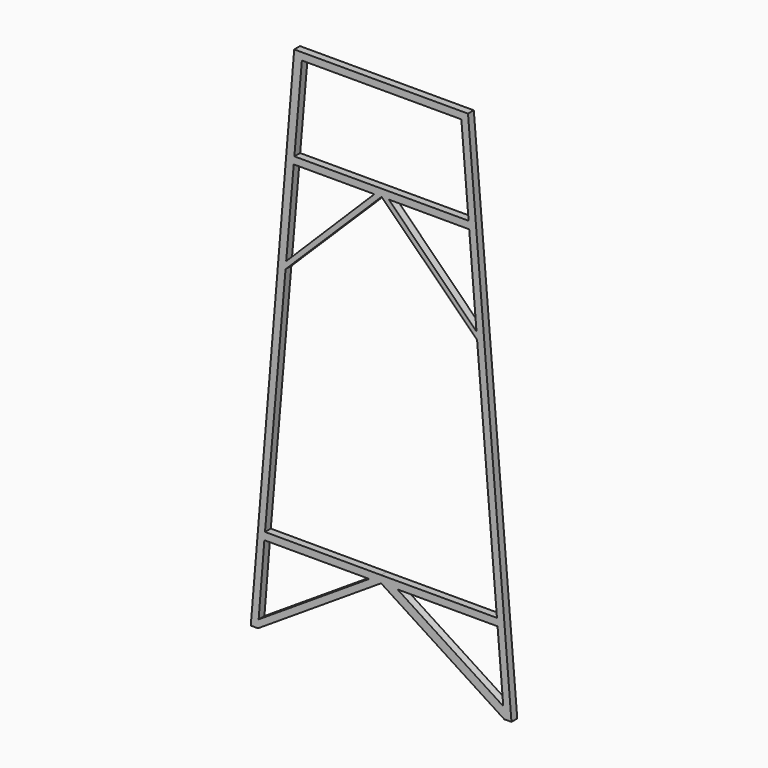
from build123d import *

# Parameters (mm, degrees)
F1_DEPTH = 25.4


# Not quite as in the source:
# - a feature names something its author has since deleted; it is built from what else it names


with BuildPart() as f1:
    # F0 (on Front) → F1 (new body)
    with BuildSketch(Plane.XZ):
        Polygon((0, 358.2734752655), (-304.8, 358.2734752655), (-457.2, -1470.5265247345), (-431.8, -1470.5265247337), (-0.1234569215, -1191.2064086248), (-1e-10, -1191.1265247345), (0.1234569213, -1191.2064086248), (431.8, -1470.5265247345), (457.2, -1470.5265247345), (304.8, 358.2734752655), align=None)
        Polygon((-429.5392940648, -1442.1890979106), (-409.5163731819, -1191.2064086248), (-41.6569560767, -1191.2064086248), align=None, mode=Mode.SUBTRACT)
        Polygon((0, -1165.7265247345), (-407.2488822076, -1164.9444627713), (-335.1759464959, -330.2), (1.7004121065, 2.7614467587), (336.7727896055, -330.2), (406.4, -1165.7265247345), align=None, mode=Mode.SUBTRACT)
        Polygon((57.3942214249, -1191.2064086248), (408.5233236575, -1191.2064086248), (428.535863163, -1431.3568826906), align=None, mode=Mode.SUBTRACT)
        Polygon((-23.6995878935, 2.7614467587), (-332.9828770612, -304.8), (-306.4276168969, 2.7614467587), align=None, mode=Mode.SUBTRACT)
        Polygon((334.6561229388, -304.8), (27.1003926271, 2.7299896004), (309.0577234879, 2.380793411), align=None, mode=Mode.SUBTRACT)
        Polygon((-277.9249521719, 332.8776175298), (281.5093551883, 332.9612130061), (306.9093551883, 28.1612130061), (-304.2345555955, 28.1613525589), align=None, mode=Mode.SUBTRACT)
    extrude(amount=F1_DEPTH)


solid = f1.part
